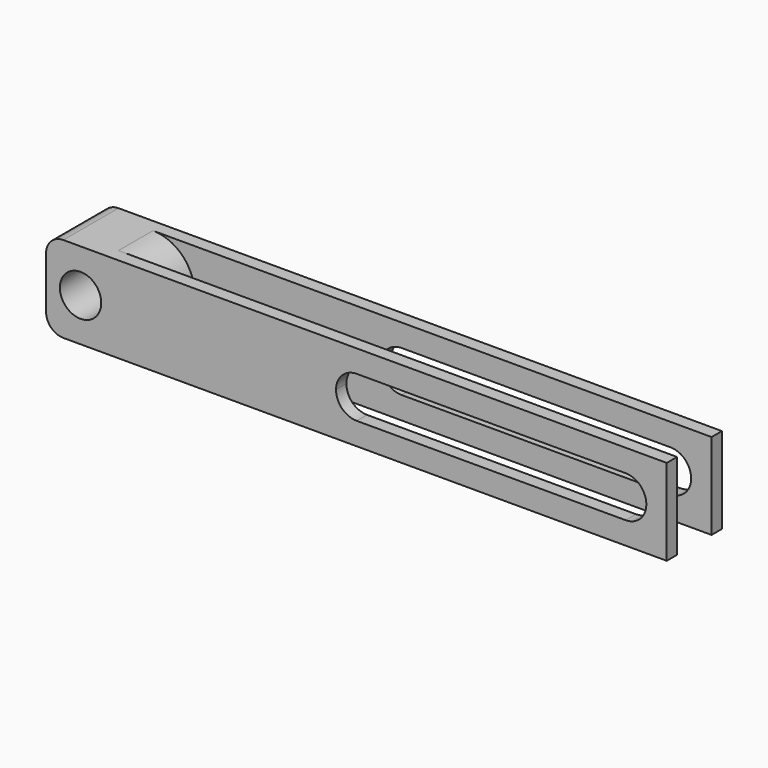
from build123d import *

# Parameters (mm, degrees)
F0_W     = 180
F0_H     = 25
F1_DEPTH = 10
F2_R     = 5
F3_R     = 6
F4_DEPTH = 12.5
F5_W     = 90
F5_H     = 12
F6_DEPTH = 12.5
F7_R     = 5.99999
F8_W     = 12.5
F8_H     = 26.6679223076
F9_DEPTH = 150
F10_R    = 12


# Not quite as in the source:
# - a fillet or chamfer is up to 0.001 mm smaller than in the source, because OpenCascade refuses the exact size


with BuildPart() as f1:
    # F0 (on Front) → F1 (new body, symmetric)
    with BuildSketch(Plane.XZ):
        with Locations((0, 12.5)):
            Rectangle(F0_W, F0_H)
    extrude(amount=F1_DEPTH, both=True)

    # F2
    f2_edges = [f1.edges().sort_by_distance(p)[0] for p in [
        (-90, 0, 25),
        (-90, 0, 0),
    ]]
    fillet(f2_edges, radius=F2_R)

    # F3 (on Front) → F4 (cut, symmetric)
    with BuildSketch(Plane.XZ):
        with Locations((-80, 12.5)):
            Circle(F3_R)
    extrude(amount=F4_DEPTH, both=True, mode=Mode.SUBTRACT)

    # F5 (on Front) → F6 (cut, symmetric)
    with BuildSketch(Plane.XZ):
        with Locations((39.0828225685, 12.5)):
            Rectangle(F5_W, F5_H)
    extrude(amount=F6_DEPTH, both=True, mode=Mode.SUBTRACT)

    # F7 (radius 6 in the source; OpenCascade refuses exactly that, so slightly less here)
    f7_edges = [f1.edges().sort_by_distance(p)[0] for p in [
        (-5.917177, 0, 6.5),
        (-5.917177, 0, 18.5),
        (84.082823, 0, 18.5),
        (84.082823, 0, 6.5),
    ]]
    fillet(f7_edges, radius=F7_R)

    # F8 (on face) → F9 (cut)
    with BuildSketch(Plane.YZ.offset(90)):
        with Locations((0, 13.3339611538)):
            Rectangle(F8_W, F8_H)
    extrude(amount=-F9_DEPTH, mode=Mode.SUBTRACT)

    # F10
    f10_edges = [f1.edges().sort_by_distance(p)[0] for p in [
        (-60, 0, 25),
        (-60, 0, 0),
    ]]
    fillet(f10_edges, radius=F10_R)


solid = f1.part
